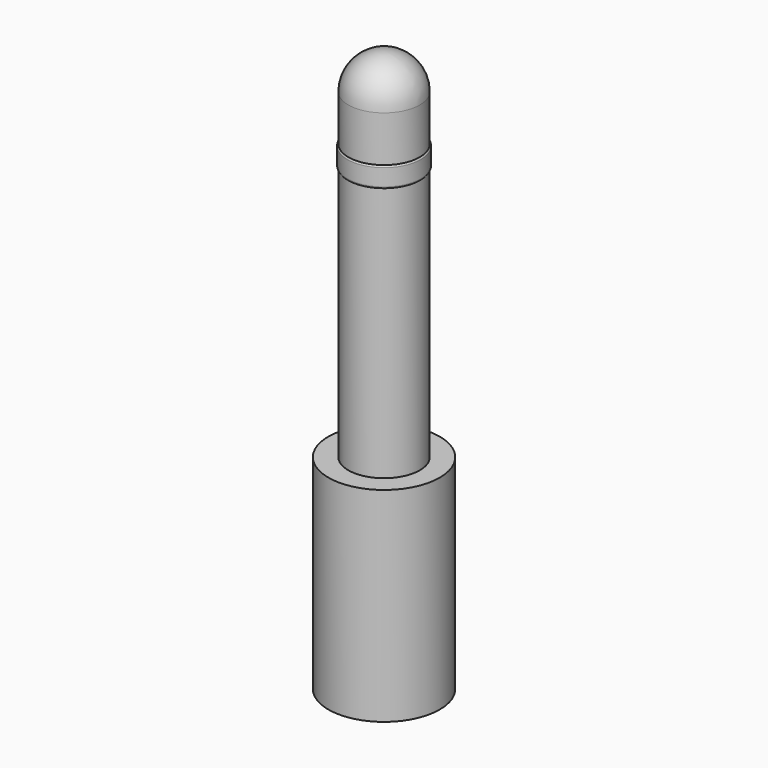
from build123d import *

# Parameters (mm, degrees)
F0_R     = 2.725
F1_DEPTH = 10
F2_R     = 1.75
F3_DEPTH = 12.5
F4_R     = 1.8
F4_R_2   = 1.75
F5_DEPTH = 1
F6_R     = 1.75
F7_DEPTH = 4
F9_R     = 1.75


# Not quite as in the source:
# - a fillet or chamfer that OpenCascade refuses, or shapes differently, is made with other operations: its cross-section is extruded or revolved along the edge and cut away or added


with BuildPart() as f1:
    # F0 (on Top) → F1 (new body)
    with BuildSketch(Plane.XY):
        Circle(F0_R)
    extrude(amount=F1_DEPTH)

    # F2 (on face) → F3 (join)
    with BuildSketch(Plane.XY.offset(10)):
        Circle(F2_R)
    extrude(amount=F3_DEPTH)

    # F4 (on face) → F5 (join)
    with BuildSketch(Plane.XY.offset(22.5)):
        Circle(F4_R)
        Circle(F4_R_2, mode=Mode.SUBTRACT)
        Circle(F4_R_2)
    extrude(amount=F5_DEPTH)

    # F6 (on face) → F7 (join)
    with BuildSketch(Plane.XY.offset(23.5)):
        Circle(F6_R)
    extrude(amount=F7_DEPTH)

    # F8: fillet of radius 0.1 on 2 edges, made by hand

    # F8_s1 → F8_t2 (revolve, cut)
    with BuildSketch(Plane.XZ):
        with BuildLine():
            ThreePointArc((1.8, 23.4133974596), (1.7866025404, 23.4633974596), (1.75, 23.5))
            Line((1.75, 23.5), (1.8, 23.5))
            Line((1.8, 23.5), (1.8, 23.4133974596))
        make_face()
    revolve(axis=Axis((0, 0, 23.5), (0, 0, 1)), mode=Mode.SUBTRACT)

    # F8_s3 → F8_t4 (revolve, cut)
    with BuildSketch(Plane.XZ):
        with BuildLine():
            ThreePointArc((1.8, 22.5866025404), (1.7866025404, 22.5366025404), (1.75, 22.5))
            Line((1.75, 22.5), (1.8, 22.5))
            Line((1.8, 22.5), (1.8, 22.5866025404))
        make_face()
    revolve(axis=Axis((0, 0, 22.5), (0, 0, 1)), mode=Mode.SUBTRACT)

    # F9
    f9_edges = [f1.edges().sort_by_distance(p)[0] for p in [
        (-1.75, 0, 27.5),
    ]]
    fillet(f9_edges, radius=F9_R)


solid = f1.part
